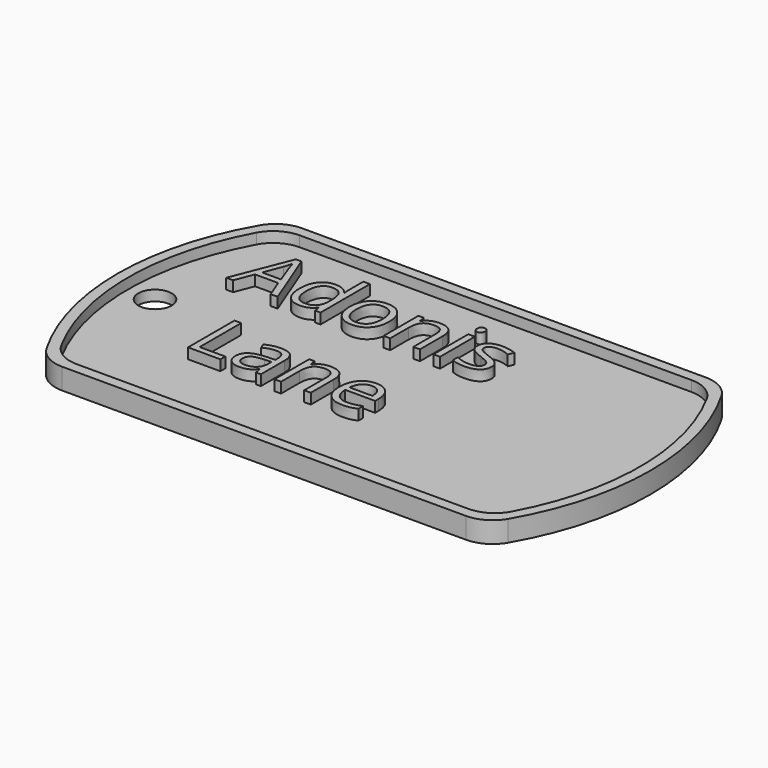
from build123d import *

# Parameters (mm, degrees)
F1_DEPTH     = 1
F3_DEPTH     = 1
F4_R         = 1.5875
F5_DEPTH     = 1
F6_TEXT_SIZE = 7.7459019443
F7_DEPTH     = 1


# Not quite as in the source:
# - Text() gives the source's letters only with a copy of the font that has no kerning and outlines rounded to 1/6400 em; it was checked with that copy


with BuildPart() as f1:
    # F0 (on Top) → F1 (new body)
    with BuildSketch(Plane.XY):
        with BuildLine():
            ThreePointArc((-19.2474145991, 14.2875), (-20.8349145991, 13.862130657), (-21.9970452561, 12.7))
            ThreePointArc((-21.9970452561, 12.7), (-25.4, 0), (-21.9970452561, -12.7))
            ThreePointArc((-21.9970452561, -12.7), (-20.8349145991, -13.862130657), (-19.2474145991, -14.2875))
            Line((-19.2474145991, -14.2875), (19.2474145991, -14.2875))
            ThreePointArc((19.2474145991, -14.2875), (20.8349145991, -13.862130657), (21.9970452561, -12.7))
            ThreePointArc((21.9970452561, -12.7), (25.4, 0), (21.9970452561, 12.7))
            ThreePointArc((21.9970452561, 12.7), (20.8349145991, 13.862130657), (19.2474145991, 14.2875))
            Line((19.2474145991, 14.2875), (-19.2474145991, 14.2875))
        make_face()
    extrude(amount=F1_DEPTH)

    # F2 (on face) → F3 (join)
    with BuildSketch(Plane.XY.offset(1)):
        with BuildLine():
            Line((19.2474145991, 14.2875), (-19.2474145991, 14.2875))
            ThreePointArc((-19.2474145991, 14.2875), (-20.8349145991, 13.862130657), (-21.9970452561, 12.7))
            ThreePointArc((-21.9970452561, 12.7), (-25.4, 0), (-21.9970452561, -12.7))
            ThreePointArc((-21.9970452561, -12.7), (-20.8349145991, -13.862130657), (-19.2474145991, -14.2875))
            Line((-19.2474145991, -14.2875), (19.2474145991, -14.2875))
            ThreePointArc((19.2474145991, -14.2875), (20.8349145991, -13.862130657), (21.9970452561, -12.7))
            ThreePointArc((21.9970452561, -12.7), (25.4, 0), (21.9970452561, 12.7))
            ThreePointArc((21.9970452561, 12.7), (20.8349145991, 13.862130657), (19.2474145991, 14.2875))
        make_face()
        with BuildLine():
            ThreePointArc((-21.4526124879, 11.6252061249), (-20.2856017842, 12.8404540819), (-18.6611352482, 13.2875))
            Line((-18.6611352482, 13.2875), (18.6611352482, 13.2875))
            ThreePointArc((18.6611352482, 13.2875), (20.2856017842, 12.8404540819), (21.4526124879, 11.6252061249))
            ThreePointArc((21.4526124879, 11.6252061249), (24.4, 0), (21.4526124879, -11.6252061249))
            ThreePointArc((21.4526124879, -11.6252061249), (20.2856017842, -12.8404540819), (18.6611352482, -13.2875))
            Line((18.6611352482, -13.2875), (-18.6611352482, -13.2875))
            ThreePointArc((-18.6611352482, -13.2875), (-20.2856017842, -12.8404540819), (-21.4526124879, -11.6252061249))
            ThreePointArc((-21.4526124879, -11.6252061249), (-24.4, 0), (-21.4526124879, 11.6252061249))
        make_face(mode=Mode.SUBTRACT)
    extrude(amount=F3_DEPTH)

    # F4 (on face) → F5 (cut)
    with BuildSketch(Plane.XY.offset(1)):
        with Locations((-21.821282804, 0)):
            Circle(F4_R)
    extrude(amount=-F5_DEPTH, mode=Mode.SUBTRACT)

    # F6 (on face) → F7 (join)
    with BuildSketch(Plane.XY.offset(1)):
        with Locations((-18.6611352482, 4.5354506001)):
            Text('Adonis', F6_TEXT_SIZE, font='Open Sans', text_align=(TextAlign.LEFT, TextAlign.BOTTOM))
        with Locations((-14.6356868315, -5.9989760442)):
            Text('Lane', F6_TEXT_SIZE, font='Open Sans', text_align=(TextAlign.LEFT, TextAlign.BOTTOM))
    extrude(amount=F7_DEPTH)


solid = f1.part
